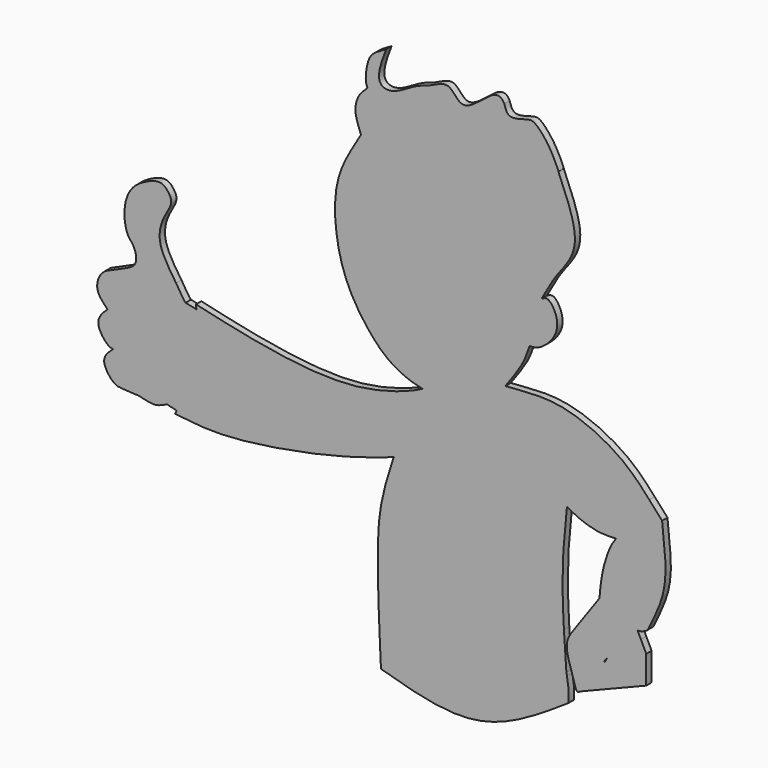
from build123d import *

# Parameters (mm, degrees)
F1_DEPTH = 3.81
F2_DEPTH = 3.81


with BuildPart() as f1:
    # F0 (on Front) → F1 (new body)
    with BuildSketch(Plane.XZ):
        with BuildLine():
            add(Edge.make_bspline(
                [(50.1290946422, 110.5438844654), (51.272035479, 111.1901077173), (54.1100535657, 112.794734324), (59.4558930701, 104.7353770997), (59.2289849467, 94.2858657595), (49.2972169564, 84.9083295298), (45.0674410109, 84.8145253424), (43.380182889, 84.777106841)],
                knots=[0, 0, 0, 0, 0.1373516627, 0.3410557137, 0.5737682339, 0.8299760984, 1, 1, 1, 1], degree=3))
            add(Edge.make_bspline(
                [(50.1290946422, 110.5438844654), (52.1482236562, 114.2951675613), (54.1673526702, 118.0464506571), (56.5864330348, 121.8042468352)],
                knots=[0, 0, 0, 0, 0.2036114651, 0.2036114651, 0.2036114651, 0.2036114651], degree=3))
            add(Edge.make_bspline(
                [(57.4488764691, 123.1179583028), (57.2019259765, 123.5959691837), (56.4778996137, 125.0247164516), (49.1186499887, 126.5153706182), (46.2596656535, 127.3285861627), (45.4135531483, 126.1757167799), (46.3510554616, 124.8991771403), (49.2194839715, 124.8823270308), (54.3016148881, 123.984783479), (55.8846693538, 122.4714216752), (56.5864330348, 121.8042468352)],
                knots=[0, 0, 0, 0, 0.1004902133, 0.3027808809, 0.4279694996, 0.4989610496, 0.5788034455, 0.7029470003, 0.8706775381, 1, 1, 1, 1], degree=3))
            add(Edge.make_bspline(
                [(57.4488764691, 123.1179583028), (57.8938486363, 123.7823848185), (58.3527692291, 124.4470384798), (58.8278462098, 125.1119552429)],
                knots=[0.2273337572, 0.2273337572, 0.2273337572, 0.2273337572, 0.2633194932, 0.2633194932, 0.2633194932, 0.2633194932], degree=3))
            add(Edge.make_bspline(
                [(60.1365069133, 126.8907462802), (59.130965886, 127.4562552247), (56.5698922703, 128.8846030135), (46.4060416373, 131.2356309245), (44.3987266175, 131.0187722363), (43.8069221748, 129.3435211667), (45.2921740659, 129.3821369465), (48.6540538623, 128.518765949), (54.4171695825, 127.6717602376), (57.3868137635, 125.9510797908), (58.8278462098, 125.1119552429)],
                knots=[0, 0, 0, 0, 0.1348386918, 0.3462396331, 0.4341645786, 0.5041260168, 0.5693290536, 0.6925155731, 0.8519880215, 1, 1, 1, 1], degree=3))
            add(Edge.make_bspline(
                [(60.1365069133, 126.8907462802), (61.0472579344, 128.0986513061), (61.9972827432, 129.3161065213), (62.9234595104, 130.5756827593)],
                knots=[0.2953866222, 0.2953866222, 0.2953866222, 0.2953866222, 0.3605872943, 0.3605872943, 0.3605872943, 0.3605872943], degree=3))
            add(Edge.make_bspline(
                [(44.0770084167, 133.888798739), (47.620722691, 134.2068131), (54.4659253271, 134.7303608915), (60.2322971244, 132.0188735382), (62.9234595104, 130.5756827593)],
                knots=[0, 0, 0, 0, 0.5146744175, 1, 1, 1, 1], degree=3))
            add(Edge.make_bspline(
                [(-32.0832874497, 166.1449426185), (-30.4350654655, 165.9413362541), (-26.2407214403, 165.4232051127), (-15.3137454014, 170.79853628), (-3.3266166752, 180.0229162527), (0.5497782421, 161.1091657967), (17.0252170187, 169.9751462319), (25.0199386016, 175.8597918731), (31.6361296689, 165.9343013645), (34.0150666268, 159.2136127579), (34.3123654621, 150.7960670315), (47.6595750238, 157.7772883891), (61.7981272539, 155.7902187189), (51.0050060469, 140.5526300558), (46.270803039, 135.9989434139), (44.0770084167, 133.888798739)],
                knots=[0, 0, 0, 0, 0.0560663648, 0.1426759409, 0.2231108716, 0.3062719495, 0.3995873002, 0.4707151626, 0.545342333, 0.6140623622, 0.6694347099, 0.7560442549, 0.831242726, 0.9217991287, 1, 1, 1, 1], degree=3))
            add(Edge.make_bspline(
                [(-32.0832874497, 166.1449426185), (-33.673663014, 166.5899953759), (-36.5512875113, 168.0673320498), (-40.410157576, 169.1536422736), (-41.6374491014, 170.5611861717)],
                knots=[0, 0, 0, 0, 0.4842893325, 1, 1, 1, 1], degree=3))
            add(Edge.make_bspline(
                [(-52.2278530762, 159.1355215947), (-50.5004615876, 161.748322356), (-47.280294596, 166.6190507478), (-43.4247617053, 169.312555789), (-41.6374491014, 170.5611861717)],
                knots=[0, 0, 0, 0, 0.5364291644, 1, 1, 1, 1], degree=3))
            add(Edge.make_bspline(
                [(-17.285336041, 43.6668989448), (-19.2842683439, 44.101077168), (-24.2887691332, 45.2032122718), (-38.7387732723, 51.4921134295), (-53.9309399961, 69.9425041242), (-63.5275512603, 88.9583291613), (-67.8889858783, 113.3184856487), (-65.9173580764, 137.2303786533), (-56.5365406772, 151.7575360103), (-52.2278530762, 159.1355215947)],
                knots=[0, 0, 0, 0, 0.0842967385, 0.2106210337, 0.3687493557, 0.5193012937, 0.6789979183, 0.8362312804, 1, 1, 1, 1], degree=3))
            add(Edge.make_bspline(
                [(-17.285336041, 43.6668989448), (-16.7202272838, 42.4787478391), (-15.0480789076, 39.0372567577), (0.9189579472, 34.8791365791), (26.6478490447, 38.5062583646), (29.9629954068, 54.8849427335), (29.7064728279, 58.6249198215), (29.6108503264, 60.0184606893)],
                knots=[0, 0, 0, 0, 0.1218373973, 0.3564423951, 0.6486196963, 0.8691174317, 1, 1, 1, 1], degree=3))
            add(Edge.make_bspline(
                [(29.6108503264, 60.0184606893), (29.6108503264, 60.1160750006), (29.6108503264, 60.213689312), (29.6108503264, 60.3113036233)],
                knots=[0, 0, 0, 0, 0.292842934, 0.292842934, 0.292842934, 0.292842934], degree=3))
            add(Edge.make_bspline(
                [(43.380182889, 84.777106841), (42.331152269, 81.6231686908), (39.925969254, 74.3919226964), (33.3299744442, 65.3880817347), (29.6108503264, 60.3113036233)],
                knots=[0, 0, 0, 0, 0.4361541777, 1, 1, 1, 1], degree=3))
        make_face()
        with BuildLine():
            add(Edge.make_bspline(
                [(-47.4406605837, 143.1240672493), (-49.8072227563, 143.083201782), (-54.9559720259, 138.1684585492), (-54.950749402, 129.8831583126), (-53.8820720623, 123.0468468699), (-46.9936805201, 115.8780450133), (-40.9662505814, 124.5453915342), (-40.4800915747, 130.4370839468), (-41.0207288883, 138.9079995292), (-45.2493318554, 143.1619068098), (-47.4406605837, 143.1240672493)],
                knots=[0, 0, 0, 0, 0.1295993794, 0.2597301523, 0.3821395271, 0.504894115, 0.6334772889, 0.7484989831, 0.8799968805, 1, 1, 1, 1], degree=3))
        make_face(mode=Mode.SUBTRACT)
        with BuildLine():
            add(Edge.make_bspline(
                [(-53.5846208733, 144.28311286), (-53.2614130923, 144.1423849511), (-52.3104533153, 143.7283275284), (-48.645138687, 146.2435555394), (-42.7414833496, 149.4443644288), (-40.2548438409, 150.1028988624), (-39.2214268355, 150.376577729)],
                knots=[0, 0, 0, 0, 0.1380713805, 0.4062412385, 0.7532411115, 1, 1, 1, 1], degree=3))
            add(Edge.make_bspline(
                [(-53.5846208733, 144.28311286), (-53.6928352381, 144.5860154138), (-54.1517302073, 145.8705071563), (-48.7726407378, 148.4247012109), (-44.6620218109, 150.376577729)],
                knots=[0, 0, 0, 0, 0.235815104, 1, 1, 1, 1], degree=3))
            add(Edge.make_bspline(
                [(-44.6620218109, 150.376577729), (-42.6932952192, 151.3111816547), (-39.6753591412, 152.7438716572), (-37.9295673746, 152.0598756256), (-37.2410125198, 151.0744138464), (-38.4678916344, 150.6420999861), (-39.2214268355, 150.376577729)],
                knots=[0, 0, 0, 0, 0.4047702984, 0.6204878281, 0.7669079395, 1, 1, 1, 1], degree=3))
        make_face(mode=Mode.SUBTRACT)
        with BuildLine():
            add(Edge.make_bspline(
                [(-15.649987888, 58.1498962712), (-15.7312997028, 58.3509772701), (-11.3227979526, 58.1356942285), (-6.7758956778, 61.5926489621), (-5.6858021479, 59.5436913756), (-4.3152880864, 57.3024170344), (-7.7123768995, 57.0921642917), (-10.4460490672, 56.7913518318), (-15.558887603, 57.9246087609), (-15.649987888, 58.1498962712)],
                knots=[0, 0, 0, 0, 0.1545236461, 0.3398064745, 0.4431023124, 0.5523242773, 0.6733242989, 0.8268745048, 1, 1, 1, 1], degree=3))
        make_face(mode=Mode.SUBTRACT)
        with BuildLine():
            add(Edge.make_bspline(
                [(-33.1750559463, 66.5078263921), (-32.9270893364, 65.814716603), (-32.6661751298, 63.3133645891), (-48.7249464744, 73.2658540563), (-36.2044501837, 82.3014349231), (-35.2742334521, 82.1792142366)],
                knots=[0.3979764529, 0.3979764529, 0.3979764529, 0.3979764529, 0.4638162222, 0.7391100879, 1, 1, 1, 1], degree=3))
            add(Edge.make_bspline(
                [(-35.2742334521, 82.1792142366), (-34.7744935407, 82.1135536728), (-35.7645460383, 80.7437414743), (-36.3271305142, 78.7609748037)],
                knots=[0, 0, 0, 0, 0.1401577687, 0.1401577687, 0.1401577687, 0.1401577687], degree=3))
            add(Edge.make_bspline(
                [(-36.3271305142, 78.7609748037), (-36.5534970136, 77.9631711498), (-37.2719731838, 73.8622133079), (-33.9336600077, 68.6282566443), (-33.1750559463, 66.5078263921)],
                knots=[0.1401577687, 0.1401577687, 0.1401577687, 0.1401577687, 0.1965528967, 0.3979764529, 0.3979764529, 0.3979764529, 0.3979764529], degree=3))
        make_face(mode=Mode.SUBTRACT)
        with BuildLine():
            add(Edge.make_bspline(
                [(1.2022150673, 82.9508526668), (0.9110680763, 83.2469431661), (1.2539612316, 84.3813393102), (1.7697807993, 87.1175853627), (4.6523209699, 87.0705285139), (8.5154615935, 84.8098073207), (11.7233437864, 84.4151117302), (14.0449502959, 79.8190197425), (13.4119547066, 76.1983575261), (12.8135183763, 72.463911043), (10.9971560988, 74.82507477), (11.6760636977, 76.8192162592), (10.9022215695, 79.7737009338), (10.2357149638, 81.3553431078), (5.5244494942, 82.5535658969), (1.7095210527, 82.4349329178), (1.2022150673, 82.9508526668)],
                knots=[0, 0, 0, 0, 0.0492059345, 0.1151320022, 0.1787581534, 0.2675535529, 0.3412154086, 0.429936325, 0.5152055619, 0.5818473736, 0.6364032668, 0.6986443448, 0.7700359082, 0.8218671731, 0.9142616415, 1, 1, 1, 1], degree=3))
        make_face(mode=Mode.SUBTRACT)
        with BuildLine():
            add(Edge.make_bspline(
                [(-21.7461024981, 134.4257941396), (-22.5291069458, 131.1998349238), (-24.3481931797, 123.7052440338), (-35.2730642309, 105.2437829352), (-36.1344705836, 103.3362503633), (-35.6699248451, 100.0568384543), (-32.0431860786, 96.8272151182), (-31.5177497308, 95.3578672556), (-31.3090932408, 94.7743732341)],
                knots=[0, 0, 0, 0, 0.2332442899, 0.5418762028, 0.6377238481, 0.7530488319, 0.9019330045, 1, 1, 1, 1], degree=3))
            add(Edge.make_bspline(
                [(-21.7461024981, 134.4257941396), (-22.5228176535, 129.4119066194), (-23.9841728578, 119.9784990566), (-29.1900419331, 109.1561620003), (-29.3701506284, 105.0629559958), (-29.4431305354, 103.4043920203)],
                knots=[0, 0, 0, 0, 0.4029115193, 0.7580601995, 1, 1, 1, 1], degree=3))
            add(Edge.make_bspline(
                [(-29.4431305354, 103.4043920203), (-27.7326819485, 101.227451191), (-26.0222333616, 99.0505103617), (-24.3117847747, 96.8735695324)],
                knots=[0, 0, 0, 0, 8.3055614912, 8.3055614912, 8.3055614912, 8.3055614912], degree=3))
            Line((-24.3117847747, 96.8735695324), (-31.3090932408, 94.7743732341))
        make_face(mode=Mode.SUBTRACT)
        with BuildLine():
            add(Edge.make_bspline(
                [(42.8111087081, 115.667431163), (42.488536201, 115.444964508), (41.8843848282, 115.0283030379), (42.9051919615, 114.8396680526), (43.7538424008, 114.8712978708), (44.8911572957, 114.976704363), (46.0577758447, 114.9153700075), (48.1925432372, 114.036866302), (48.8745203782, 113.6225287638), (49.5388567239, 113.6716091453), (49.4774725338, 113.9028358222), (49.4515853749, 114.0003495585)],
                knots=[0, 0, 0, 0, 0.1083543571, 0.2029386639, 0.3181215753, 0.4408103352, 0.5714952436, 0.7492807005, 0.858369136, 0.9402709285, 1, 1, 1, 1], degree=3))
            add(Edge.make_bspline(
                [(42.8111087081, 115.667431163), (43.7644208212, 115.7749179197), (45.8461954904, 116.0096397954), (48.1842187601, 114.7066552417), (49.4515853749, 114.0003495585)],
                knots=[0, 0, 0, 0, 0.4579324205, 1, 1, 1, 1], degree=3))
        make_face(mode=Mode.SUBTRACT)
        with BuildLine():
            add(Edge.make_bspline(
                [(45.7247809175, 119.759947051), (45.1809022443, 119.7983749894), (44.0308148853, 119.6617058738), (44.1250130918, 121.8598297453), (47.9906962224, 121.2030831883), (50.2909633812, 120.5806389056), (51.6011470046, 119.6611351197), (52.17347276, 118.2173306248), (50.4832712065, 117.9037875013), (49.3333749225, 119.1512505835), (47.3800165177, 119.362359281), (46.3187345262, 119.7179810504), (45.7247809175, 119.759947051)],
                knots=[0, 0, 0, 0, 0.0919038298, 0.1741418848, 0.314694825, 0.438190681, 0.5331098271, 0.6138328152, 0.6968999651, 0.7946559994, 0.8996345802, 1, 1, 1, 1], degree=3))
        make_face(mode=Mode.SUBTRACT)
        with BuildLine():
            add(Edge.make_bspline(
                [(-0.5928435735, 133.8170865973), (-0.9881429716, 133.4951278709), (-1.7664060856, 132.861257437), (-0.5683058684, 131.1365497874), (1.3319321943, 133.0888100472), (2.1534546975, 133.7667453233), (3.5901456703, 135.3891369133), (6.5494669763, 136.6400025622), (11.5378763278, 135.5541735009), (14.0249076728, 134.3771987721), (15.2084645508, 133.8170865973)],
                knots=[0, 0, 0, 0, 0.0940613013, 0.185187333, 0.306409369, 0.3960728682, 0.5105497543, 0.6534660493, 0.8350874662, 1, 1, 1, 1], degree=3))
            add(Edge.make_bspline(
                [(-0.5928435735, 133.8170865973), (1.4165850955, 135.7945971833), (5.7618326577, 141.5827057395), (19.063534972, 134.2340865459), (21.5038602655, 130.7235598497), (22.4650623971, 129.2161212808)],
                knots=[0, 0, 0, 0, 0.3242596956, 0.7253937013, 1, 1, 1, 1], degree=3))
            add(Edge.make_bspline(
                [(15.2084645508, 133.8170865973), (15.4207090738, 133.6722439145), (16.0727714049, 133.2272550115), (19.3845451557, 130.4406276347), (20.4868096692, 128.9259843311), (21.8170540092, 128.0758402817), (22.2508228341, 128.8391303226), (22.4650623971, 129.2161212808)],
                knots=[0, 0, 0, 0, 0.15034224, 0.4618847645, 0.6805029855, 0.8421995845, 1, 1, 1, 1], degree=3))
        make_face(mode=Mode.SUBTRACT)
        with BuildLine():
            add(Edge.make_bspline(
                [(8.7010575055, 154.2983448735), (8.1880224009, 154.1504565314), (7.1523421678, 153.8519096459), (6.57756081, 152.3364318542), (6.7033003627, 150.9664032256), (6.9364599699, 150.966749653), (7.0038889448, 150.9668498386)],
                knots=[0, 0, 0, 0, 0.3058456508, 0.6174203131, 0.8893592402, 1, 1, 1, 1], degree=3))
            add(Edge.make_bspline(
                [(7.0038889448, 150.9668498386), (7.2213554044, 150.7754139053), (7.8219643018, 150.246697316), (10.9561335594, 150.2742924783), (14.1118805013, 149.0840063103), (16.927360202, 147.0991600034), (19.6132876617, 145.0712211907), (20.5600508242, 142.2066535233), (23.3782298508, 143.5848846761), (22.0403181729, 145.7573431211), (20.3806641818, 148.8702799232), (17.4351275502, 150.9342894888), (14.2532359968, 153.6849449752), (10.3465719629, 154.8782915367), (9.1638701636, 154.4614590021), (8.7010575055, 154.2983448735)],
                knots=[0, 0, 0, 0, 0.0450489812, 0.1244183538, 0.2099518454, 0.2954007521, 0.3805147425, 0.4519841715, 0.5160494038, 0.5815603885, 0.6687209444, 0.7555657357, 0.8512192221, 0.941779384, 1, 1, 1, 1], degree=3))
        make_face(mode=Mode.SUBTRACT)
        with BuildLine():
            add(Edge.make_bspline(
                [(57.4488764691, 123.1179583028), (57.2019259765, 123.5959691837), (56.4778996137, 125.0247164516), (49.1186499887, 126.5153706182), (46.2596656535, 127.3285861627), (45.4135531483, 126.1757167799), (46.3510554616, 124.8991771403), (49.2194839715, 124.8823270308), (54.3016148881, 123.984783479), (55.8846693538, 122.4714216752), (56.5864330348, 121.8042468352)],
                knots=[0, 0, 0, 0, 0.1004902133, 0.3027808809, 0.4279694996, 0.4989610496, 0.5788034455, 0.7029470003, 0.8706775381, 1, 1, 1, 1], degree=3))
            add(Edge.make_bspline(
                [(56.5864330348, 121.8042468352), (56.8682743893, 122.2420588156), (57.1555446959, 122.6799592047), (57.4488764691, 123.1179583028)],
                knots=[0.2036114651, 0.2036114651, 0.2036114651, 0.2036114651, 0.2273337572, 0.2273337572, 0.2273337572, 0.2273337572], degree=3))
        make_face()
        with BuildLine():
            add(Edge.make_bspline(
                [(29.6108503264, 60.3113036233), (31.8536355668, 60.4746532479), (35.2647954062, 60.723099541), (41.0300356213, 61.1927812645), (43.2150031501, 61.3064438267)],
                knots=[0, 0, 0, 0, 0.1507315045, 0.229254788, 0.229254788, 0.229254788, 0.229254788], degree=3))
            add(Edge.make_bspline(
                [(29.6108503264, 60.0184606893), (29.6108503264, 60.1160750006), (29.6108503264, 60.213689312), (29.6108503264, 60.3113036233)],
                knots=[0, 0, 0, 0, 0.292842934, 0.292842934, 0.292842934, 0.292842934], degree=3))
            add(Edge.make_bspline(
                [(-17.285336041, 43.6668989448), (-16.7202272838, 42.4787478391), (-15.0480789076, 39.0372567577), (0.9189579472, 34.8791365791), (26.6478490447, 38.5062583646), (29.9629954068, 54.8849427335), (29.7064728279, 58.6249198215), (29.6108503264, 60.0184606893)],
                knots=[0, 0, 0, 0, 0.1218373973, 0.3564423951, 0.6486196963, 0.8691174317, 1, 1, 1, 1], degree=3))
            add(Edge.make_bspline(
                [(-24.8652586351, 40.1660025391), (-21.5100045662, 41.5000238277), (-19.3969411039, 42.5834128123), (-17.285336041, 43.6668989448)],
                knots=[0.8685611959, 0.8685611959, 0.8685611959, 0.8685611959, 1, 1, 1, 1], degree=3))
            add(Edge.make_bspline(
                [(-24.8652586351, 40.1660025391), (-24.3795003919, 38.7022637334), (-23.0415356151, 34.6705648548), (-8.1382907268, 26.1875139155), (-2.0423290254, 26.2323328302), (0.5270009031, 26.2512231357)],
                knots=[0, 0, 0, 0, 0.2479825511, 0.6830391933, 1, 1, 1, 1], degree=3))
            add(Edge.make_bspline(
                [(0.5270009031, 26.2512231357), (-1.0773265021, 17.6723431708), (-4.4148268602, -0.1677960336), (-9.6927375089, -30.5118855403), (-6.0703026349, -61.4799158123), (-3.2473125148, -77.7002017445), (-3.6818282777, -78.239197683)],
                knots=[0, 0, 0, 0, 0.2489554093, 0.5171779955, 0.7991042426, 0.9779843861, 0.9779843861, 0.9779843861, 0.9779843861], degree=3))
            add(Edge.make_bspline(
                [(-3.6818282777, -78.239197683), (2.940720686, -77.392588893), (9.8847031633, -75.9934750876), (16.4839384121, -74.2720243176)],
                knots=[0.3419059811, 0.3419059811, 0.3419059811, 0.3419059811, 0.4852230953, 0.4852230953, 0.4852230953, 0.4852230953], degree=3))
            add(Edge.make_bspline(
                [(21.5391564169, 27.5029533069), (19.5961358971, 20.5065575017), (15.642216339, 6.2689965136), (13.3081204278, -17.4561234594), (10.7008694881, -34.8852258535), (12.7336702861, -53.0941595724), (15.1972201767, -66.9980992006), (16.4839384121, -74.2720243176)],
                knots=[0, 0, 0, 0, 0.2078360694, 0.4228276205, 0.6075099932, 0.7942879381, 1, 1, 1, 1], degree=3))
            add(Edge.make_bspline(
                [(43.2150031501, 61.3064438267), (43.4232076872, 57.4107776436), (43.8813165859, 48.9702202439), (34.6212051861, 34.9203733822), (25.8584739162, 29.9501748768), (21.5391564169, 27.5029533069)],
                knots=[0, 0, 0, 0, 0.3053599404, 0.6571625588, 1, 1, 1, 1], degree=3))
        make_face()
        with BuildLine():
            add(Edge.make_bspline(
                [(60.1365069133, 126.8907462802), (59.130965886, 127.4562552247), (56.5698922703, 128.8846030135), (46.4060416373, 131.2356309245), (44.3987266175, 131.0187722363), (43.8069221748, 129.3435211667), (45.2921740659, 129.3821369465), (48.6540538623, 128.518765949), (54.4171695825, 127.6717602376), (57.3868137635, 125.9510797908), (58.8278462098, 125.1119552429)],
                knots=[0, 0, 0, 0, 0.1348386918, 0.3462396331, 0.4341645786, 0.5041260168, 0.5693290536, 0.6925155731, 0.8519880215, 1, 1, 1, 1], degree=3))
            add(Edge.make_bspline(
                [(58.8278462098, 125.1119552429), (59.0229089122, 125.3849645992), (59.4521644898, 125.9775726186), (59.8949692696, 126.5704012825), (60.1365069133, 126.8907462802)],
                knots=[0.2633194932, 0.2633194932, 0.2633194932, 0.2633194932, 0.2780949405, 0.2953866222, 0.2953866222, 0.2953866222, 0.2953866222], degree=3))
        make_face()
        with BuildLine():
            add(Edge.make_bspline(
                [(43.2150031501, 61.3064438267), (48.4401508317, 61.5782573276), (66.0005024414, 61.5832401891), (95.7636273566, 47.3430541695), (106.4626040298, 35.4034006987), (111.1927043758, 30.1247875435)],
                knots=[0.229254788, 0.229254788, 0.229254788, 0.229254788, 0.417035955, 0.7422670864, 1, 1, 1, 1], degree=3))
            add(Edge.make_bspline(
                [(43.2150031501, 61.3064438267), (43.4232076872, 57.4107776436), (43.8813165859, 48.9702202439), (34.6212051861, 34.9203733822), (25.8584739162, 29.9501748768), (21.5391564169, 27.5029533069)],
                knots=[0, 0, 0, 0, 0.3053599404, 0.6571625588, 1, 1, 1, 1], degree=3))
            add(Edge.make_bspline(
                [(21.5391564169, 27.5029533069), (19.5961358971, 20.5065575017), (15.642216339, 6.2689965136), (13.3081204278, -17.4561234594), (10.7008694881, -34.8852258535), (12.7336702861, -53.0941595724), (15.1972201767, -66.9980992006), (16.4839384121, -74.2720243176)],
                knots=[0, 0, 0, 0, 0.2078360694, 0.4228276205, 0.6075099932, 0.7942879381, 1, 1, 1, 1], degree=3))
            add(Edge.make_bspline(
                [(16.4839384121, -74.2720243176), (20.3625000818, -73.2602778469), (35.3902954554, -68.7709398477), (52.1530179094, -60.3287254609), (59.620820296, -53.3242681414), (62.8313386985, -50.4619171764)],
                knots=[0.4852230953, 0.4852230953, 0.4852230953, 0.4852230953, 0.5694547137, 0.8219229724, 1, 1, 1, 1], degree=3))
            add(Edge.make_bspline(
                [(64.5389668057, 11.4656303012), (63.3748265165, 0.3064383398), (61.4220697103, -18.4122575563), (62.287799682, -41.0500536507), (62.8313386985, -50.4619171764)],
                knots=[0, 0, 0, 0, 0.4604650729, 0.7723951429, 0.7723951429, 0.7723951429, 0.7723951429], degree=3))
            add(Edge.make_bspline(
                [(75.8550337667, 6.3237607461), (74.3834843926, 6.8082039827), (71.0848490184, 7.8941353318), (66.8722754029, 10.1925551608), (64.5389668057, 11.4656303012)],
                knots=[0, 0, 0, 0, 0.4461085288, 1, 1, 1, 1], degree=3))
            add(Edge.make_bspline(
                [(75.8550337667, 6.3237607461), (78.138402547, 5.6585682821), (83.0171267745, 4.2372951973), (89.159649525, 4.4782474568), (92.4273131878, 4.6064278437)],
                knots=[0, 0, 0, 0, 0.468025794, 1, 1, 1, 1], degree=3))
            add(Edge.make_bspline(
                [(92.4273131878, 4.6064278437), (91.342466474, 3.1335851015), (88.5783054323, -0.6191796688), (84.0709596257, -15.0383368222), (83.3397115148, -23.895992676), (82.9819728285, -28.2293046148)],
                knots=[0, 0, 0, 0, 0.2481027973, 0.632159436, 1, 1, 1, 1], degree=3))
            add(Edge.make_bspline(
                [(82.9819728285, -28.2293046148), (83.4995641642, -28.9780183464), (84.9975164458, -31.1448580229), (96.0536906937, -35.2814774619), (101.8352665265, -36.541261956), (104.5599279186, -37.1349558334)],
                knots=[0, 0, 0, 0, 0.2182310217, 0.6315786882, 1, 1, 1, 1], degree=3))
            add(Edge.make_bspline(
                [(104.5599279186, -37.1349558334), (105.0982510511, -37.2182459054), (106.3905387436, -37.4181903781), (109.7227855306, -35.794897638), (110.266045236, -35.2321785017), (110.4541867971, -35.0372977555)],
                knots=[0, 0, 0, 0, 0.3182071437, 0.7638816737, 1, 1, 1, 1], degree=3))
            add(Edge.make_bspline(
                [(118.4851817836, 22.0337749543), (119.3754228801, 14.3698993978), (121.0294797592, 0.1305139826), (119.5337068165, -16.4683134199), (113.5947812208, -28.6143096974), (110.4541867971, -35.0372977555)],
                knots=[0, 0, 0, 0, 0.3544948596, 0.6586470378, 1, 1, 1, 1], degree=3))
            add(Edge.make_bspline(
                [(111.1927043758, 30.1247875435), (113.6235301784, 27.4277833471), (116.054355981, 24.7307791507), (118.4851817836, 22.0337749543)],
                knots=[0, 0, 0, 0, 10.8924153181, 10.8924153181, 10.8924153181, 10.8924153181], degree=3))
        make_face()
        with BuildLine():
            add(Edge.make_bspline(
                [(44.0770084167, 133.888798739), (47.620722691, 134.2068131), (54.4659253271, 134.7303608915), (60.2322971244, 132.0188735382), (62.9234595104, 130.5756827593)],
                knots=[0, 0, 0, 0, 0.5146744175, 1, 1, 1, 1], degree=3))
            add(Edge.make_bspline(
                [(62.9234595104, 130.5756827593), (66.2760058002, 135.1350582403), (74.0011565693, 148.1233621218), (59.4754859859, 176.4057449335), (59.7861630943, 177.0831170136), (59.8167241552, 177.1497495683)],
                knots=[0.3605872943, 0.3605872943, 0.3605872943, 0.3605872943, 0.5965986899, 0.9603177328, 1, 1, 1, 1], degree=3))
            add(Edge.make_bspline(
                [(29.0284052889, 201.0991242813), (29.6672057348, 198.8351882083), (31.1095129596, 193.7235897806), (42.0140968081, 197.7035374795), (46.5260398695, 197.9804624009), (55.1584196576, 187.8674459448), (58.2615246957, 180.7279088794), (59.8167241552, 177.1497495683)],
                knots=[0, 0, 0, 0, 0.1688314284, 0.3811938305, 0.5237170795, 0.7612987857, 1, 1, 1, 1], degree=3))
            add(Edge.make_bspline(
                [(-37.9073243902, 206.4650942791), (-38.7920737972, 204.2438868818), (-40.6840649567, 199.4939489608), (-43.5235863216, 187.8976672548), (-34.222742532, 184.8349373366), (-21.4132432464, 194.2923049701), (-12.8945960357, 195.8643059095), (-1.6607526108, 202.9519683896), (5.1642418135, 186.7896620028), (20.958020447, 204.3519579746), (27.1369852105, 204.052767749), (28.4561573893, 201.9927471681), (29.0284052889, 201.0991242813)],
                knots=[0, 0, 0, 0, 0.0921575307, 0.1970741454, 0.2827218193, 0.4107692548, 0.5128288495, 0.6178088046, 0.724609981, 0.8669515582, 0.9422844928, 1, 1, 1, 1], degree=3))
            add(Edge.make_bspline(
                [(-37.9073243902, 206.4650942791), (-40.6682895645, 204.960767825), (-45.6913525976, 202.2239254077), (-48.6082245091, 197.1330241949), (-50.0163775464, 187.53372225), (-49.0083493426, 184.843570506), (-48.6151765749, 183.7942998578)],
                knots=[0, 0, 0, 0, 0.2839945684, 0.5166753393, 0.8114833555, 1, 1, 1, 1], degree=3))
            add(Edge.make_bspline(
                [(-48.6151765749, 183.7942998578), (-48.2644996992, 182.5715525854), (-47.4397778102, 179.6958955055), (-43.273669353, 172.9480817142), (-42.0835554781, 171.2119600029), (-41.6374491014, 170.5611861717)],
                knots=[0, 0, 0, 0, 0.3162216927, 0.7436901883, 1, 1, 1, 1], degree=3))
            add(Edge.make_bspline(
                [(-32.0832874497, 166.1449426185), (-33.673663014, 166.5899953759), (-36.5512875113, 168.0673320498), (-40.410157576, 169.1536422736), (-41.6374491014, 170.5611861717)],
                knots=[0, 0, 0, 0, 0.4842893325, 1, 1, 1, 1], degree=3))
            add(Edge.make_bspline(
                [(-32.0832874497, 166.1449426185), (-30.4350654655, 165.9413362541), (-26.2407214403, 165.4232051127), (-15.3137454014, 170.79853628), (-3.3266166752, 180.0229162527), (0.5497782421, 161.1091657967), (17.0252170187, 169.9751462319), (25.0199386016, 175.8597918731), (31.6361296689, 165.9343013645), (34.0150666268, 159.2136127579), (34.3123654621, 150.7960670315), (47.6595750238, 157.7772883891), (61.7981272539, 155.7902187189), (51.0050060469, 140.5526300558), (46.270803039, 135.9989434139), (44.0770084167, 133.888798739)],
                knots=[0, 0, 0, 0, 0.0560663648, 0.1426759409, 0.2231108716, 0.3062719495, 0.3995873002, 0.4707151626, 0.545342333, 0.6140623622, 0.6694347099, 0.7560442549, 0.831242726, 0.9217991287, 1, 1, 1, 1], degree=3))
        make_face()
        with BuildLine():
            add(Edge.make_bspline(
                [(-24.8652586351, 40.1660025391), (-24.3795003919, 38.7022637334), (-23.0415356151, 34.6705648548), (-8.1382907268, 26.1875139155), (-2.0423290254, 26.2323328302), (0.5270009031, 26.2512231357)],
                knots=[0, 0, 0, 0, 0.2479825511, 0.6830391933, 1, 1, 1, 1], degree=3))
            add(Edge.make_bspline(
                [(-145.7655614105, 44.0781430585), (-130.6274797393, 40.6283540199), (-100.4503617544, 33.7469783411), (-55.3398865161, 29.9934264455), (-31.1905755559, 37.6511088064), (-24.8652586351, 40.1660025391)],
                knots=[0, 0, 0, 0, 0.3114012005, 0.6207730779, 0.8685611959, 0.8685611959, 0.8685611959, 0.8685611959], degree=3))
            add(Edge.make_bspline(
                [(-145.7655614105, 44.0781430585), (-145.6881488802, 43.2627283581), (-145.6107363499, 42.4473136577), (-145.5333238196, 41.6318989573)],
                knots=[0, 0, 0, 0, 2.4572432727, 2.4572432727, 2.4572432727, 2.4572432727], degree=3))
            add(Edge.make_bspline(
                [(-156.7360054688, -12.5161372104), (-154.2145819594, -8.2873756016), (-149.2126048885, 0.1016032932), (-142.4886120564, 13.2837005416), (-144.4059773269, 31.1355877973), (-145.5333238196, 41.6318989573)],
                knots=[0, 0, 0, 0, 0.2951900778, 0.585595397, 1, 1, 1, 1], degree=3))
            add(Edge.make_bspline(
                [(-157.6537845208, -14.445924666), (-157.3478581701, -13.8026621808), (-157.0419318194, -13.1593996956), (-156.7360054688, -12.5161372104)],
                knots=[0, 0, 0, 0, 2.1369131971, 2.1369131971, 2.1369131971, 2.1369131971], degree=3))
            add(Edge.make_bspline(
                [(-157.6537845208, -14.445924666), (-148.9750479933, -15.5103634302), (-127.886004773, -18.0969144832), (-68.1302533051, -7.5013355971), (-44.1155954801, 0.6712875681), (-33.5744447389, 4.2586321541)],
                knots=[0, 0, 0, 0, 0.2817919165, 0.6847450533, 1, 1, 1, 1], degree=3))
            add(Edge.make_bspline(
                [(-33.7802285616, 3.9988264164), (-33.7192726037, 4.1009756171), (-33.6354006968, 4.1564829534), (-33.5744447389, 4.2586321541)],
                knots=[0, 0, 0, 0, 0.3314302385, 0.3314302385, 0.3314302385, 0.3314302385], degree=3))
            add(Edge.make_bspline(
                [(-33.7802285616, 3.9988264164), (-36.5566928384, -4.6272377561), (-42.3271822156, -22.5552954264), (-42.9802623892, -47.6157921782), (-42.4098692239, -67.5419533043), (-42.1347499408, -75.0031942381)],
                knots=[0, 0, 0, 0, 0.2910684217, 0.6049446591, 0.7809924038, 0.7809924038, 0.7809924038, 0.7809924038], degree=3))
            add(Edge.make_bspline(
                [(-42.1347499408, -75.0031942381), (-34.3065690543, -77.0895083277), (-23.391493998, -79.9354481629), (-8.1836263162, -78.8076144758), (-3.8882971011, -78.2654260736)],
                knots=[0, 0, 0, 0, 0.2473666468, 0.3404158417, 0.3404158417, 0.3404158417, 0.3404158417], degree=3))
            add(Edge.make_bspline(
                [(-3.8882971011, -78.2654260736), (-3.8195094087, -78.2567431794), (-3.7506862179, -78.2480002963), (-3.6818282777, -78.239197683)],
                knots=[0.3404158417, 0.3404158417, 0.3404158417, 0.3404158417, 0.3419059811, 0.3419059811, 0.3419059811, 0.3419059811], degree=3))
            add(Edge.make_bspline(
                [(0.5270009031, 26.2512231357), (-1.0773265021, 17.6723431708), (-4.4148268602, -0.1677960336), (-9.6927375089, -30.5118855403), (-6.0703026349, -61.4799158123), (-3.2473125148, -77.7002017445), (-3.6818282777, -78.239197683)],
                knots=[0, 0, 0, 0, 0.2489554093, 0.5171779955, 0.7991042426, 0.9779843861, 0.9779843861, 0.9779843861, 0.9779843861], degree=3))
        make_face()
        with BuildLine():
            add(Edge.make_bspline(
                [(-48.6151765749, 183.7942998578), (-49.2061443999, 182.6426911676), (-52.8364333659, 180.3930144581), (-57.2482954595, 170.2200884419), (-52.8986098283, 161.1688939726), (-52.2278530762, 159.1355215947)],
                knots=[0, 0, 0, 0, 0.2516779894, 0.6211962177, 1, 1, 1, 1], degree=3))
            add(Edge.make_bspline(
                [(-52.2278530762, 159.1355215947), (-50.5004615876, 161.748322356), (-47.280294596, 166.6190507478), (-43.4247617053, 169.312555789), (-41.6374491014, 170.5611861717)],
                knots=[0, 0, 0, 0, 0.5364291644, 1, 1, 1, 1], degree=3))
            add(Edge.make_bspline(
                [(-48.6151765749, 183.7942998578), (-48.2644996992, 182.5715525854), (-47.4397778102, 179.6958955055), (-43.273669353, 172.9480817142), (-42.0835554781, 171.2119600029), (-41.6374491014, 170.5611861717)],
                knots=[0, 0, 0, 0, 0.3162216927, 0.7436901883, 1, 1, 1, 1], degree=3))
        make_face()
        with BuildLine():
            add(Edge.make_bspline(
                [(16.4839384121, -74.2720243176), (20.3625000818, -73.2602778469), (35.3902954554, -68.7709398477), (52.1530179094, -60.3287254609), (59.620820296, -53.3242681414), (62.8313386985, -50.4619171764)],
                knots=[0.4852230953, 0.4852230953, 0.4852230953, 0.4852230953, 0.5694547137, 0.8219229724, 1, 1, 1, 1], degree=3))
            add(Edge.make_bspline(
                [(-3.6818282777, -78.239197683), (2.940720686, -77.392588893), (9.8847031633, -75.9934750876), (16.4839384121, -74.2720243176)],
                knots=[0.3419059811, 0.3419059811, 0.3419059811, 0.3419059811, 0.4852230953, 0.4852230953, 0.4852230953, 0.4852230953], degree=3))
            add(Edge.make_bspline(
                [(-3.6818282777, -78.239197683), (-3.73530616, -78.305534428), (-3.8119651359, -78.2846594639), (-3.8882971011, -78.2654260736)],
                knots=[0.9779843861, 0.9779843861, 0.9779843861, 0.9779843861, 1, 1, 1, 1], degree=3))
            add(Edge.make_bspline(
                [(-42.1347499408, -75.0031942381), (-34.3065690543, -77.0895083277), (-23.391493998, -79.9354481629), (-8.1836263162, -78.8076144758), (-3.8882971011, -78.2654260736)],
                knots=[0, 0, 0, 0, 0.2473666468, 0.3404158417, 0.3404158417, 0.3404158417, 0.3404158417], degree=3))
            add(Edge.make_bspline(
                [(-42.1347499408, -75.0031942381), (-41.9411339174, -80.2540649979), (-41.7127718538, -85.6540297372), (-41.4693198281, -91.1187449482)],
                knots=[0.7809924038, 0.7809924038, 0.7809924038, 0.7809924038, 0.9048865338, 0.9048865338, 0.9048865338, 0.9048865338], degree=3))
            add(Edge.make_bspline(
                [(-41.4693198281, -91.1187449482), (-34.2241922657, -93.2388308652), (-17.8735508897, -97.9520842331), (18.6792798387, -96.2654830973), (49.6482545518, -80.1509309291), (60.2555819483, -74.9805314189), (64.5239635713, -72.8971036621)],
                knots=[0, 0, 0, 0, 0.2349744242, 0.5254419557, 0.8085747703, 1, 1, 1, 1], degree=3))
            add(Edge.make_bspline(
                [(64.2276316246, -71.3515950569), (64.3272245139, -71.8668777381), (64.4268174032, -72.3821604193), (64.5239635713, -72.8971036621)],
                knots=[0, 0, 0, 0, 0.1021920967, 0.1021920967, 0.1021920967, 0.1021920967], degree=3))
            add(Edge.make_bspline(
                [(62.8313386985, -50.4619171764), (63.2279407963, -57.3294367207), (63.7277862104, -64.3405158888), (64.2276316246, -71.3515950569)],
                knots=[0.7723951429, 0.7723951429, 0.7723951429, 0.7723951429, 1, 1, 1, 1], degree=3))
        make_face()
        with BuildLine():
            add(Edge.make_bspline(
                [(-156.7360054688, -12.5161372104), (-154.2145819594, -8.2873756016), (-149.2126048885, 0.1016032932), (-142.4886120564, 13.2837005416), (-144.4059773269, 31.1355877973), (-145.5333238196, 41.6318989573)],
                knots=[0, 0, 0, 0, 0.2951900778, 0.585595397, 1, 1, 1, 1], degree=3))
            add(Edge.make_bspline(
                [(-145.5333238196, 41.6318989573), (-147.4708608552, 42.0470877022), (-149.6766043074, 42.5127718675), (-151.6141413429, 42.9279606123)],
                knots=[0, 0, 0, 0, 6.2174044074, 6.2174044074, 6.2174044074, 6.2174044074], degree=3))
            add(Edge.make_bspline(
                [(-147.3978207109, 37.4074223846), (-147.4649380726, 37.9303152921), (-147.6190565591, 39.1310100363), (-149.5229702798, 41.2868382948), (-150.9197959292, 42.383047872), (-151.6141413429, 42.9279606123)],
                knots=[0, 0, 0, 0, 0.2795250825, 0.6418604892, 1, 1, 1, 1], degree=3))
            add(Edge.make_bspline(
                [(-151.5412264819, 14.4854143051), (-151.2731458581, 14.4714214104), (-150.3664200542, 14.4240934142), (-147.4803619648, 19.6662129837), (-146.8612649506, 24.8718400598), (-147.4103851545, 37.1390560746), (-147.3989866047, 37.3825198385), (-147.3978207109, 37.4074223846)],
                knots=[0, 0, 0, 0, 0.0984582575, 0.3330141561, 0.6077660977, 0.9598805889, 1, 1, 1, 1], degree=3))
            add(Edge.make_bspline(
                [(-153.2231919182, 14.2401347261), (-153.0252150638, 14.2105292682), (-152.567428637, 14.1420718881), (-151.9127686078, 14.3611052975), (-151.5412264819, 14.4854143051)],
                knots=[0, 0, 0, 0, 0.4324655404, 1, 1, 1, 1], degree=3))
            add(Edge.make_bspline(
                [(-152.1080079791, 13.6522492628), (-152.2345903534, 13.7787877228), (-152.5583935276, 13.9720897717), (-152.9833832568, 14.1716426391), (-153.2231919182, 14.2401347261)],
                knots=[0, 0, 0, 0, 0.4647373753, 1, 1, 1, 1], degree=3))
            add(Edge.make_bspline(
                [(-161.9289218202, -11.1396595296), (-160.1310604683, -9.2882403932), (-155.3136909457, -7.5657334089), (-152.8582395195, -2.2000658374), (-151.6762720127, 5.8766736077), (-152.0156842352, 11.1468199998), (-152.1080079791, 13.6522492628)],
                knots=[0, 0, 0, 0, 0.2534602483, 0.4720946711, 0.7381478624, 1, 1, 1, 1], degree=3))
            add(Edge.make_bspline(
                [(-162.002260766, -11.170356582), (-161.9779050791, -11.1601409303), (-161.9534591378, -11.1499084747), (-161.9289218202, -11.1396595296)],
                knots=[0.9969611333, 0.9969611333, 0.9969611333, 0.9969611333, 1, 1, 1, 1], degree=3))
            add(Edge.make_bspline(
                [(-156.7360054688, -12.5161372104), (-158.3418088421, -12.1527437573), (-160.8513419648, -11.6681909299), (-161.7941919281, -11.2094909566), (-162.002260766, -11.170356582)],
                knots=[0, 0, 0, 0, 0.6757569087, 0.9291238043, 0.9291238043, 0.9291238043, 0.9291238043], degree=3))
        make_face()
        with BuildLine():
            add(Edge.make_bspline(
                [(105.0551623339, -38.2615932732), (104.8892412209, -37.8841090125), (104.7258490316, -37.5124400941), (104.5599279186, -37.1349558334)],
                knots=[0, 0, 0, 0, 1.2306782874, 1.2306782874, 1.2306782874, 1.2306782874], degree=3))
            add(Edge.make_bspline(
                [(82.9819728285, -28.2293046148), (83.4995641642, -28.9780183464), (84.9975164458, -31.1448580229), (96.0536906937, -35.2814774619), (101.8352665265, -36.541261956), (104.5599279186, -37.1349558334)],
                knots=[0, 0, 0, 0, 0.2182310217, 0.6315786882, 1, 1, 1, 1], degree=3))
            add(Edge.make_bspline(
                [(82.9819728285, -28.2293046148), (79.4879227555, -33.1486679566), (75.9938726825, -38.0680312985), (72.4998226095, -42.9873946403)],
                knots=[0, 0, 0, 0, 18.1018422934, 18.1018422934, 18.1018422934, 18.1018422934], degree=3))
            add(Edge.make_bspline(
                [(72.4998226095, -42.9873946403), (71.0751876127, -44.8444116718), (68.1238661064, -48.6914702621), (63.4756455801, -56.193850401), (64.7892577685, -61.6609378621), (65.4416076834, -64.3759355392)],
                knots=[0, 0, 0, 0, 0.3196089385, 0.6621125664, 1, 1, 1, 1], degree=3))
            add(Edge.make_bspline(
                [(65.4416076834, -64.3759355392), (66.8675097836, -68.9769697616), (68.2934118837, -73.5780039839), (69.7193139839, -78.1790382063)],
                knots=[0, 0, 0, 0, 14.4507582649, 14.4507582649, 14.4507582649, 14.4507582649], degree=3))
            add(Edge.make_bspline(
                [(69.7193139839, -78.1790382063), (69.9028088042, -78.5475504446), (70.3425013821, -79.4305840684), (71.5981818524, -78.6398051219), (72.3298351415, -78.1790382063)],
                knots=[0, 0, 0, 0, 0.4173252619, 1, 1, 1, 1], degree=3))
            add(Edge.make_bspline(
                [(72.3298351415, -78.1790382063), (84.7175015593, -73.1937570738), (97.105167977, -68.2084759414), (109.4928343948, -63.2231948089)],
                knots=[0, 0, 0, 0, 40.0595277708, 40.0595277708, 40.0595277708, 40.0595277708], degree=3))
            add(Edge.make_bspline(
                [(109.4928343948, -63.2231948089), (109.4928343948, -57.9357774192), (109.4928343948, -52.6483600294), (109.4928343948, -47.3609426397)],
                knots=[0, 0, 0, 0, 15.8622521693, 15.8622521693, 15.8622521693, 15.8622521693], degree=3))
            add(Edge.make_bspline(
                [(109.4928343948, -47.3609426397), (108.4857072729, -45.2958505345), (107.478580151, -43.2307584293), (106.4714530292, -41.1656663242)],
                knots=[0, 0, 0, 0, 6.8927638855, 6.8927638855, 6.8927638855, 6.8927638855], degree=3))
            add(Edge.make_bspline(
                [(106.4714530292, -41.1656663242), (105.9993561308, -40.1976419738), (105.5272592323, -39.2296176235), (105.0551623339, -38.2615932732)],
                knots=[6.8927638855, 6.8927638855, 6.8927638855, 6.8927638855, 10.1237884318, 10.1237884318, 10.1237884318, 10.1237884318], degree=3))
        make_face()
        with BuildLine():
            add(Edge.make_bspline(
                [(87.7388813588, -56.122947347), (86.65684804, -57.3234643296), (85.5748147211, -58.5239813122), (85.9260512866, -59.1443318447)],
                knots=[0, 0, 0, 0, 0.3840401317, 0.3840401317, 0.3840401317, 0.3840401317], degree=3))
            add(Edge.make_bspline(
                [(87.7388813588, -56.122947347), (87.1346046681, -57.1300755129), (86.5303279774, -58.1372036788), (85.9260512866, -59.1443318447)],
                knots=[7.0470184201, 7.0470184201, 7.0470184201, 7.0470184201, 10.5705276301, 10.5705276301, 10.5705276301, 10.5705276301], degree=3))
        make_face(mode=Mode.SUBTRACT)
        with BuildLine():
            add(Edge.make_bspline(
                [(-147.3978207109, 37.4074223846), (-147.4649380726, 37.9303152921), (-147.6190565591, 39.1310100363), (-149.5229702798, 41.2868382948), (-150.9197959292, 42.383047872), (-151.6141413429, 42.9279606123)],
                knots=[0, 0, 0, 0, 0.2795250825, 0.6418604892, 1, 1, 1, 1], degree=3))
            add(Edge.make_bspline(
                [(-151.6141413429, 42.9279606123), (-151.8992805654, 43.2305379051), (-152.9679493417, 44.1548308026), (-155.2483442261, 48.2651591184), (-157.0243867353, 51.0065816003)],
                knots=[0, 0, 0, 0, 0.3041244084, 1, 1, 1, 1], degree=3))
            add(Edge.make_bspline(
                [(-197.1685046067, 43.9805025363), (-191.8420889147, 46.5308693636), (-183.9030454968, 49.4381808582), (-178.8495682297, 53.4638110447), (-180.4219196602, 61.8528824741), (-185.4537722652, 65.9017175024), (-187.1929485496, 78.8246471903), (-183.4064239369, 90.1678542198), (-175.0893668564, 96.0888843798), (-165.812103776, 99.4272134109), (-161.8743385456, 95.8569747336), (-158.6624264054, 90.814744311), (-162.414811946, 84.2370897633), (-165.3378887362, 79.0315662076), (-167.014603187, 71.1040628536), (-164.6227834582, 62.4449413403), (-159.7557654654, 54.8894816786), (-157.0243867353, 51.0065816003)],
                knots=[0, 0, 0, 0, 0.0885904036, 0.1421533509, 0.2039172796, 0.2616747383, 0.3421225874, 0.4206520049, 0.493922476, 0.5627055279, 0.6121589934, 0.6651502452, 0.7255045751, 0.7828581422, 0.8462335827, 0.9143911763, 1, 1, 1, 1], degree=3))
            add(Edge.make_bspline(
                [(-197.1685046067, 43.9805025363), (-197.1730414384, 43.9765430037), (-197.1579575497, 43.9274079188), (-197.1649946586, 43.9242068825)],
                knots=[0, 0, 0, 0, 0.4864128982, 0.4864128982, 0.4864128982, 0.4864128982], degree=3))
            add(Edge.make_bspline(
                [(-197.1649946586, 43.9242068825), (-189.1175417154, 44.0797027319), (-175.5274252561, 44.342295967), (-164.2424043709, 42.8229713256), (-158.5344667044, 30.1030304716), (-164.614730584, 25.0545274808), (-166.1250241432, 24.2887388589), (-166.8907450077, 24.1825881957)],
                knots=[0, 0, 0, 0, 0.2736779723, 0.4621730057, 0.6576250259, 0.8061549454, 0.8955576254, 0.8955576254, 0.8955576254, 0.8955576254], degree=3))
            add(Edge.make_bspline(
                [(-166.8907450077, 24.1825881957), (-164.8690674412, 23.8910852633), (-160.0973115572, 23.1891894091), (-159.2543107764, 10.5543952603), (-162.2229105191, 7.0021968259), (-166.1536313067, 6.1841257401), (-167.3032974442, 6.0273279886)],
                knots=[0, 0, 0, 0, 0.1788496673, 0.421998126, 0.6051750012, 0.668839839, 0.668839839, 0.668839839, 0.668839839], degree=3))
            add(Edge.make_bspline(
                [(-167.3032974442, 6.0273279886), (-165.3910667431, 6.0184279252), (-161.1046170758, 6.001634244), (-160.4787303189, -3.1961256408), (-161.4232722377, -8.8415419348), (-164.5640328274, -11.0092737727), (-166.107416153, -12.0744695887)],
                knots=[0, 0, 0, 0, 0.2315311631, 0.5190012252, 0.7636422208, 1, 1, 1, 1], degree=3))
            Line((-166.107416153, -12.0744695887), (-178.8873385571, -12.0286653477))
            add(Edge.make_bspline(
                [(-178.8873385571, -12.0286653477), (-178.7767663102, -12.0347805148), (-177.4348402946, -12.1841074702), (-168.6896091087, -14.780835988), (-165.3375816363, -12.5693102029), (-162.002260766, -11.170356582)],
                knots=[0.1022369708, 0.1022369708, 0.1022369708, 0.1022369708, 0.1478174087, 0.5808121007, 0.9969611333, 0.9969611333, 0.9969611333, 0.9969611333], degree=3))
            add(Edge.make_bspline(
                [(-162.002260766, -11.170356582), (-161.9779050791, -11.1601409303), (-161.9534591378, -11.1499084747), (-161.9289218202, -11.1396595296)],
                knots=[0.9969611333, 0.9969611333, 0.9969611333, 0.9969611333, 1, 1, 1, 1], degree=3))
            add(Edge.make_bspline(
                [(-161.9289218202, -11.1396595296), (-160.1310604683, -9.2882403932), (-155.3136909457, -7.5657334089), (-152.8582395195, -2.2000658374), (-151.6762720127, 5.8766736077), (-152.0156842352, 11.1468199998), (-152.1080079791, 13.6522492628)],
                knots=[0, 0, 0, 0, 0.2534602483, 0.4720946711, 0.7381478624, 1, 1, 1, 1], degree=3))
            add(Edge.make_bspline(
                [(-152.1080079791, 13.6522492628), (-152.2345903534, 13.7787877228), (-152.5583935276, 13.9720897717), (-152.9833832568, 14.1716426391), (-153.2231919182, 14.2401347261)],
                knots=[0, 0, 0, 0, 0.4647373753, 1, 1, 1, 1], degree=3))
            add(Edge.make_bspline(
                [(-153.2231919182, 14.2401347261), (-153.0252150638, 14.2105292682), (-152.567428637, 14.1420718881), (-151.9127686078, 14.3611052975), (-151.5412264819, 14.4854143051)],
                knots=[0, 0, 0, 0, 0.4324655404, 1, 1, 1, 1], degree=3))
            add(Edge.make_bspline(
                [(-151.5412264819, 14.4854143051), (-151.2731458581, 14.4714214104), (-150.3664200542, 14.4240934142), (-147.4803619648, 19.6662129837), (-146.8612649506, 24.8718400598), (-147.4103851545, 37.1390560746), (-147.3989866047, 37.3825198385), (-147.3978207109, 37.4074223846)],
                knots=[0, 0, 0, 0, 0.0984582575, 0.3330141561, 0.6077660977, 0.9598805889, 1, 1, 1, 1], degree=3))
        make_face()
        with BuildLine():
            add(Edge.make_bspline(
                [(64.5239635713, -72.8971036621), (64.910111762, -74.9439615615), (65.6781452152, -79.4561378409), (65.5066657082, -83.8379736496), (65.4127706075, -86.2372860893)],
                knots=[0.1021920967, 0.1021920967, 0.1021920967, 0.1021920967, 0.5083974469, 1, 1, 1, 1], degree=3))
            add(Edge.make_bspline(
                [(-41.4693198281, -91.1187449482), (-34.2241922657, -93.2388308652), (-17.8735508897, -97.9520842331), (18.6792798387, -96.2654830973), (49.6482545518, -80.1509309291), (60.2555819483, -74.9805314189), (64.5239635713, -72.8971036621)],
                knots=[0, 0, 0, 0, 0.2349744242, 0.5254419557, 0.8085747703, 1, 1, 1, 1], degree=3))
            add(Edge.make_bspline(
                [(-41.4693198281, -91.1187449482), (-41.2824218209, -95.3140042814), (-41.0866303547, -99.5474251195), (-40.8908388885, -103.7808459577)],
                knots=[0.9048865338, 0.9048865338, 0.9048865338, 0.9048865338, 1, 1, 1, 1], degree=3))
            add(Edge.make_bspline(
                [(-40.8908388885, -103.7808459577), (-22.4517153131, -109.1262393763), (14.9023853186, -119.9549733376), (48.4335909568, -97.5715625143), (65.4127706075, -86.2372860893)],
                knots=[0, 0, 0, 0, 0.4936305054, 1, 1, 1, 1], degree=3))
        make_face()
        with BuildLine():
            Line((-179.1238087613, -12.02781782), (-178.8873385571, -12.0286653477))
            add(Edge.make_bspline(
                [(-179.1238087613, -12.02781782), (-179.0514717803, -12.0240635404), (-178.9747965332, -12.0238285088), (-178.8873385571, -12.0286653477)],
                knots=[0.06618477, 0.06618477, 0.06618477, 0.06618477, 0.1022369708, 0.1022369708, 0.1022369708, 0.1022369708], degree=3))
        make_face()
        with BuildLine():
            add(Edge.make_bspline(
                [(-179.1238087613, -12.02781782), (-179.0514717803, -12.0240635404), (-178.9747965332, -12.0238285088), (-178.8873385571, -12.0286653477)],
                knots=[0.06618477, 0.06618477, 0.06618477, 0.06618477, 0.1022369708, 0.1022369708, 0.1022369708, 0.1022369708], degree=3))
            Line((-178.8873385571, -12.0286653477), (-166.107416153, -12.0744695887))
            add(Edge.make_bspline(
                [(-167.3032974442, 6.0273279886), (-165.3910667431, 6.0184279252), (-161.1046170758, 6.001634244), (-160.4787303189, -3.1961256408), (-161.4232722377, -8.8415419348), (-164.5640328274, -11.0092737727), (-166.107416153, -12.0744695887)],
                knots=[0, 0, 0, 0, 0.2315311631, 0.5190012252, 0.7636422208, 1, 1, 1, 1], degree=3))
            add(Edge.make_bspline(
                [(-167.3032974442, 6.0273279886), (-167.3063826204, 6.0269072154), (-167.3094687751, 6.0264868325), (-167.3125559076, 6.0260668397)],
                knots=[0.668839839, 0.668839839, 0.668839839, 0.668839839, 0.6690106862, 0.6690106862, 0.6690106862, 0.6690106862], degree=3))
            add(Edge.make_bspline(
                [(-167.4619102164, 6.0061506711), (-167.3686517772, 6.0108515471), (-167.33988096, 6.0175383581), (-167.3125559076, 6.0260668397)],
                knots=[0.9281415531, 0.9281415531, 0.9281415531, 0.9281415531, 1, 1, 1, 1], degree=3))
            add(Edge.make_bspline(
                [(-167.4619102164, 6.0061506711), (-173.4532484321, 5.223171909), (-183.0244881506, 5.8682478706), (-192.594059741, 6.5128412284)],
                knots=[0.6717519663, 0.6717519663, 0.6717519663, 0.6717519663, 1, 1, 1, 1], degree=3))
            add(Edge.make_bspline(
                [(-188.9903742816, -11.3271794099), (-190.0241741969, -11.3895610877), (-192.7891645814, -10.737182954), (-200.6907749986, -0.5991539994), (-195.2162752204, 4.2701540421), (-192.594059741, 6.5128412284)],
                knots=[0, 0, 0, 0, 0.2311306505, 0.6280298854, 1, 1, 1, 1], degree=3))
            add(Edge.make_bspline(
                [(-188.9903742816, -11.3271794099), (-188.7063090691, -11.4230769499), (-188.4222438566, -11.4669852219), (-188.1381786442, -11.5628827619)],
                knots=[0, 0, 0, 0, 0.8841908587, 0.8841908587, 0.8841908587, 0.8841908587], degree=3))
            Line((-188.1381786442, -11.5628827619), (-179.5182079077, -12.0744695887))
            add(Edge.make_bspline(
                [(-179.5182079077, -12.0744695887), (-179.3747810615, -12.0534625463), (-179.2566052713, -12.0347099409), (-179.1238087613, -12.02781782)],
                knots=[0, 0, 0, 0, 0.06618477, 0.06618477, 0.06618477, 0.06618477], degree=3))
        make_face()
        with BuildLine():
            add(Edge.make_bspline(
                [(-197.1649946586, 43.9242068825), (-189.1175417154, 44.0797027319), (-175.5274252561, 44.342295967), (-164.2424043709, 42.8229713256), (-158.5344667044, 30.1030304716), (-164.614730584, 25.0545274808), (-166.1250241432, 24.2887388589), (-166.8907450077, 24.1825881957)],
                knots=[0, 0, 0, 0, 0.2736779723, 0.4621730057, 0.6576250259, 0.8061549454, 0.8955576254, 0.8955576254, 0.8955576254, 0.8955576254], degree=3))
            add(Edge.make_bspline(
                [(-197.1649946586, 43.9242068825), (-198.1837659611, 43.1306044916), (-200.5915481049, 41.2549905423), (-203.1741531952, 32.5932950717), (-198.4305495089, 27.7911806128), (-195.9133020317, 25.2428837259)],
                knots=[0, 0, 0, 0, 0.2560834628, 0.6052321926, 1, 1, 1, 1], degree=3))
            add(Edge.make_bspline(
                [(-195.9133020317, 25.2428837259), (-187.3126141597, 24.9275531613), (-178.7161049955, 24.6215522395), (-170.1154171235, 24.3062216749)],
                knots=[0, 0, 0, 0, 25.8148833336, 25.8148833336, 25.8148833336, 25.8148833336], degree=3))
            add(Edge.make_bspline(
                [(-166.8907450077, 24.1825881957), (-167.7852786544, 24.0585804218), (-168.950347889, 24.1824010483), (-170.1154171235, 24.3062216749)],
                knots=[0.8955576254, 0.8955576254, 0.8955576254, 0.8955576254, 1, 1, 1, 1], degree=3))
        make_face()
        with BuildLine():
            add(Edge.make_bspline(
                [(-195.9133020317, 25.2428837259), (-187.3126141597, 24.9275531613), (-178.7161049955, 24.6215522395), (-170.1154171235, 24.3062216749)],
                knots=[0, 0, 0, 0, 25.8148833336, 25.8148833336, 25.8148833336, 25.8148833336], degree=3))
            add(Edge.make_bspline(
                [(-192.594059741, 6.5128412284), (-193.3934342973, 6.5104551018), (-195.9456493002, 6.7553333131), (-204.112089787, 17.2274428066), (-198.5940718268, 22.6743413654), (-195.9133020317, 25.2428837259)],
                knots=[0, 0, 0, 0, 0.2108336963, 0.6130626551, 1, 1, 1, 1], degree=3))
            add(Edge.make_bspline(
                [(-192.594059741, 6.5128412284), (-180.6294446336, 6.2160278046), (-168.6664593881, 5.9454329895), (-167.4619102164, 6.0061506711)],
                knots=[0, 0, 0, 0, 0.9281415531, 0.9281415531, 0.9281415531, 0.9281415531], degree=3))
            add(Edge.make_bspline(
                [(-167.3125559076, 6.0260668397), (-167.3620896123, 6.0193279649), (-167.4118750773, 6.0126895194), (-167.4619102164, 6.0061506711)],
                knots=[0.6690106862, 0.6690106862, 0.6690106862, 0.6690106862, 0.6717519663, 0.6717519663, 0.6717519663, 0.6717519663], degree=3))
            add(Edge.make_bspline(
                [(-167.3032974442, 6.0273279886), (-167.3063826204, 6.0269072154), (-167.3094687751, 6.0264868325), (-167.3125559076, 6.0260668397)],
                knots=[0.668839839, 0.668839839, 0.668839839, 0.668839839, 0.6690106862, 0.6690106862, 0.6690106862, 0.6690106862], degree=3))
            add(Edge.make_bspline(
                [(-166.8907450077, 24.1825881957), (-164.8690674412, 23.8910852633), (-160.0973115572, 23.1891894091), (-159.2543107764, 10.5543952603), (-162.2229105191, 7.0021968259), (-166.1536313067, 6.1841257401), (-167.3032974442, 6.0273279886)],
                knots=[0, 0, 0, 0, 0.1788496673, 0.421998126, 0.6051750012, 0.668839839, 0.668839839, 0.668839839, 0.668839839], degree=3))
            add(Edge.make_bspline(
                [(-166.8907450077, 24.1825881957), (-167.7852786544, 24.0585804218), (-168.950347889, 24.1824010483), (-170.1154171235, 24.3062216749)],
                knots=[0.8955576254, 0.8955576254, 0.8955576254, 0.8955576254, 1, 1, 1, 1], degree=3))
        make_face()
        with BuildLine():
            add(Edge.make_bspline(
                [(-192.594059741, 6.5128412284), (-180.6294446336, 6.2160278046), (-168.6664593881, 5.9454329895), (-167.4619102164, 6.0061506711)],
                knots=[0, 0, 0, 0, 0.9281415531, 0.9281415531, 0.9281415531, 0.9281415531], degree=3))
            add(Edge.make_bspline(
                [(-167.4619102164, 6.0061506711), (-173.4532484321, 5.223171909), (-183.0244881506, 5.8682478706), (-192.594059741, 6.5128412284)],
                knots=[0.6717519663, 0.6717519663, 0.6717519663, 0.6717519663, 1, 1, 1, 1], degree=3))
        make_face()
    extrude(amount=-F1_DEPTH)

    # F0 (on Front) → F2 (join)
    with BuildSketch(Plane.XZ):
        with BuildLine():
            add(Edge.make_bspline(
                [(-47.4406605837, 143.1240672493), (-49.8072227563, 143.083201782), (-54.9559720259, 138.1684585492), (-54.950749402, 129.8831583126), (-53.8820720623, 123.0468468699), (-46.9936805201, 115.8780450133), (-40.9662505814, 124.5453915342), (-40.4800915747, 130.4370839468), (-41.0207288883, 138.9079995292), (-45.2493318554, 143.1619068098), (-47.4406605837, 143.1240672493)],
                knots=[0, 0, 0, 0, 0.1295993794, 0.2597301523, 0.3821395271, 0.504894115, 0.6334772889, 0.7484989831, 0.8799968805, 1, 1, 1, 1], degree=3))
        make_face()
        with BuildLine():
            add(Edge.make_bspline(
                [(-0.5928435735, 133.8170865973), (1.4165850955, 135.7945971833), (5.7618326577, 141.5827057395), (19.063534972, 134.2340865459), (21.5038602655, 130.7235598497), (22.4650623971, 129.2161212808)],
                knots=[0, 0, 0, 0, 0.3242596956, 0.7253937013, 1, 1, 1, 1], degree=3))
            add(Edge.make_bspline(
                [(-0.5928435735, 133.8170865973), (-0.9881429716, 133.4951278709), (-1.7664060856, 132.861257437), (-0.5683058684, 131.1365497874), (1.3319321943, 133.0888100472), (2.1534546975, 133.7667453233), (3.5901456703, 135.3891369133), (6.5494669763, 136.6400025622), (11.5378763278, 135.5541735009), (14.0249076728, 134.3771987721), (15.2084645508, 133.8170865973)],
                knots=[0, 0, 0, 0, 0.0940613013, 0.185187333, 0.306409369, 0.3960728682, 0.5105497543, 0.6534660493, 0.8350874662, 1, 1, 1, 1], degree=3))
            add(Edge.make_bspline(
                [(15.2084645508, 133.8170865973), (15.4207090738, 133.6722439145), (16.0727714049, 133.2272550115), (19.3845451557, 130.4406276347), (20.4868096692, 128.9259843311), (21.8170540092, 128.0758402817), (22.2508228341, 128.8391303226), (22.4650623971, 129.2161212808)],
                knots=[0, 0, 0, 0, 0.15034224, 0.4618847645, 0.6805029855, 0.8421995845, 1, 1, 1, 1], degree=3))
        make_face()
        with BuildLine():
            add(Edge.make_bspline(
                [(-21.7461024981, 134.4257941396), (-22.5228176535, 129.4119066194), (-23.9841728578, 119.9784990566), (-29.1900419331, 109.1561620003), (-29.3701506284, 105.0629559958), (-29.4431305354, 103.4043920203)],
                knots=[0, 0, 0, 0, 0.4029115193, 0.7580601995, 1, 1, 1, 1], degree=3))
            add(Edge.make_bspline(
                [(-21.7461024981, 134.4257941396), (-22.5291069458, 131.1998349238), (-24.3481931797, 123.7052440338), (-35.2730642309, 105.2437829352), (-36.1344705836, 103.3362503633), (-35.6699248451, 100.0568384543), (-32.0431860786, 96.8272151182), (-31.5177497308, 95.3578672556), (-31.3090932408, 94.7743732341)],
                knots=[0, 0, 0, 0, 0.2332442899, 0.5418762028, 0.6377238481, 0.7530488319, 0.9019330045, 1, 1, 1, 1], degree=3))
            Line((-31.3090932408, 94.7743732341), (-24.3117847747, 96.8735695324))
            add(Edge.make_bspline(
                [(-29.4431305354, 103.4043920203), (-27.7326819485, 101.227451191), (-26.0222333616, 99.0505103617), (-24.3117847747, 96.8735695324)],
                knots=[0, 0, 0, 0, 8.3055614912, 8.3055614912, 8.3055614912, 8.3055614912], degree=3))
        make_face()
        with BuildLine():
            add(Edge.make_bspline(
                [(-35.2742334521, 82.1792142366), (-34.7744935407, 82.1135536728), (-35.7645460383, 80.7437414743), (-36.3271305142, 78.7609748037)],
                knots=[0, 0, 0, 0, 0.1401577687, 0.1401577687, 0.1401577687, 0.1401577687], degree=3))
            add(Edge.make_bspline(
                [(-33.1750559463, 66.5078263921), (-32.9270893364, 65.814716603), (-32.6661751298, 63.3133645891), (-48.7249464744, 73.2658540563), (-36.2044501837, 82.3014349231), (-35.2742334521, 82.1792142366)],
                knots=[0.3979764529, 0.3979764529, 0.3979764529, 0.3979764529, 0.4638162222, 0.7391100879, 1, 1, 1, 1], degree=3))
            add(Edge.make_bspline(
                [(-36.3271305142, 78.7609748037), (-36.5534970136, 77.9631711498), (-37.2719731838, 73.8622133079), (-33.9336600077, 68.6282566443), (-33.1750559463, 66.5078263921)],
                knots=[0.1401577687, 0.1401577687, 0.1401577687, 0.1401577687, 0.1965528967, 0.3979764529, 0.3979764529, 0.3979764529, 0.3979764529], degree=3))
        make_face()
        with BuildLine():
            add(Edge.make_bspline(
                [(1.2022150673, 82.9508526668), (0.9110680763, 83.2469431661), (1.2539612316, 84.3813393102), (1.7697807993, 87.1175853627), (4.6523209699, 87.0705285139), (8.5154615935, 84.8098073207), (11.7233437864, 84.4151117302), (14.0449502959, 79.8190197425), (13.4119547066, 76.1983575261), (12.8135183763, 72.463911043), (10.9971560988, 74.82507477), (11.6760636977, 76.8192162592), (10.9022215695, 79.7737009338), (10.2357149638, 81.3553431078), (5.5244494942, 82.5535658969), (1.7095210527, 82.4349329178), (1.2022150673, 82.9508526668)],
                knots=[0, 0, 0, 0, 0.0492059345, 0.1151320022, 0.1787581534, 0.2675535529, 0.3412154086, 0.429936325, 0.5152055619, 0.5818473736, 0.6364032668, 0.6986443448, 0.7700359082, 0.8218671731, 0.9142616415, 1, 1, 1, 1], degree=3))
        make_face()
        with BuildLine():
            add(Edge.make_bspline(
                [(45.7247809175, 119.759947051), (45.1809022443, 119.7983749894), (44.0308148853, 119.6617058738), (44.1250130918, 121.8598297453), (47.9906962224, 121.2030831883), (50.2909633812, 120.5806389056), (51.6011470046, 119.6611351197), (52.17347276, 118.2173306248), (50.4832712065, 117.9037875013), (49.3333749225, 119.1512505835), (47.3800165177, 119.362359281), (46.3187345262, 119.7179810504), (45.7247809175, 119.759947051)],
                knots=[0, 0, 0, 0, 0.0919038298, 0.1741418848, 0.314694825, 0.438190681, 0.5331098271, 0.6138328152, 0.6968999651, 0.7946559994, 0.8996345802, 1, 1, 1, 1], degree=3))
        make_face()
        with BuildLine():
            add(Edge.make_bspline(
                [(42.8111087081, 115.667431163), (43.7644208212, 115.7749179197), (45.8461954904, 116.0096397954), (48.1842187601, 114.7066552417), (49.4515853749, 114.0003495585)],
                knots=[0, 0, 0, 0, 0.4579324205, 1, 1, 1, 1], degree=3))
            add(Edge.make_bspline(
                [(42.8111087081, 115.667431163), (42.488536201, 115.444964508), (41.8843848282, 115.0283030379), (42.9051919615, 114.8396680526), (43.7538424008, 114.8712978708), (44.8911572957, 114.976704363), (46.0577758447, 114.9153700075), (48.1925432372, 114.036866302), (48.8745203782, 113.6225287638), (49.5388567239, 113.6716091453), (49.4774725338, 113.9028358222), (49.4515853749, 114.0003495585)],
                knots=[0, 0, 0, 0, 0.1083543571, 0.2029386639, 0.3181215753, 0.4408103352, 0.5714952436, 0.7492807005, 0.858369136, 0.9402709285, 1, 1, 1, 1], degree=3))
        make_face()
        with BuildLine():
            add(Edge.make_bspline(
                [(-15.649987888, 58.1498962712), (-15.7312997028, 58.3509772701), (-11.3227979526, 58.1356942285), (-6.7758956778, 61.5926489621), (-5.6858021479, 59.5436913756), (-4.3152880864, 57.3024170344), (-7.7123768995, 57.0921642917), (-10.4460490672, 56.7913518318), (-15.558887603, 57.9246087609), (-15.649987888, 58.1498962712)],
                knots=[0, 0, 0, 0, 0.1545236461, 0.3398064745, 0.4431023124, 0.5523242773, 0.6733242989, 0.8268745048, 1, 1, 1, 1], degree=3))
        make_face()
        with BuildLine():
            add(Edge.make_bspline(
                [(-53.5846208733, 144.28311286), (-53.6928352381, 144.5860154138), (-54.1517302073, 145.8705071563), (-48.7726407378, 148.4247012109), (-44.6620218109, 150.376577729)],
                knots=[0, 0, 0, 0, 0.235815104, 1, 1, 1, 1], degree=3))
            add(Edge.make_bspline(
                [(-53.5846208733, 144.28311286), (-53.2614130923, 144.1423849511), (-52.3104533153, 143.7283275284), (-48.645138687, 146.2435555394), (-42.7414833496, 149.4443644288), (-40.2548438409, 150.1028988624), (-39.2214268355, 150.376577729)],
                knots=[0, 0, 0, 0, 0.1380713805, 0.4062412385, 0.7532411115, 1, 1, 1, 1], degree=3))
            add(Edge.make_bspline(
                [(-44.6620218109, 150.376577729), (-42.6932952192, 151.3111816547), (-39.6753591412, 152.7438716572), (-37.9295673746, 152.0598756256), (-37.2410125198, 151.0744138464), (-38.4678916344, 150.6420999861), (-39.2214268355, 150.376577729)],
                knots=[0, 0, 0, 0, 0.4047702984, 0.6204878281, 0.7669079395, 1, 1, 1, 1], degree=3))
        make_face()
        with BuildLine():
            add(Edge.make_bspline(
                [(7.0038889448, 150.9668498386), (7.2213554044, 150.7754139053), (7.8219643018, 150.246697316), (10.9561335594, 150.2742924783), (14.1118805013, 149.0840063103), (16.927360202, 147.0991600034), (19.6132876617, 145.0712211907), (20.5600508242, 142.2066535233), (23.3782298508, 143.5848846761), (22.0403181729, 145.7573431211), (20.3806641818, 148.8702799232), (17.4351275502, 150.9342894888), (14.2532359968, 153.6849449752), (10.3465719629, 154.8782915367), (9.1638701636, 154.4614590021), (8.7010575055, 154.2983448735)],
                knots=[0, 0, 0, 0, 0.0450489812, 0.1244183538, 0.2099518454, 0.2954007521, 0.3805147425, 0.4519841715, 0.5160494038, 0.5815603885, 0.6687209444, 0.7555657357, 0.8512192221, 0.941779384, 1, 1, 1, 1], degree=3))
            add(Edge.make_bspline(
                [(8.7010575055, 154.2983448735), (8.1880224009, 154.1504565314), (7.1523421678, 153.8519096459), (6.57756081, 152.3364318542), (6.7033003627, 150.9664032256), (6.9364599699, 150.966749653), (7.0038889448, 150.9668498386)],
                knots=[0, 0, 0, 0, 0.3058456508, 0.6174203131, 0.8893592402, 1, 1, 1, 1], degree=3))
        make_face()
    extrude(amount=-F2_DEPTH)


solid = f1.part
